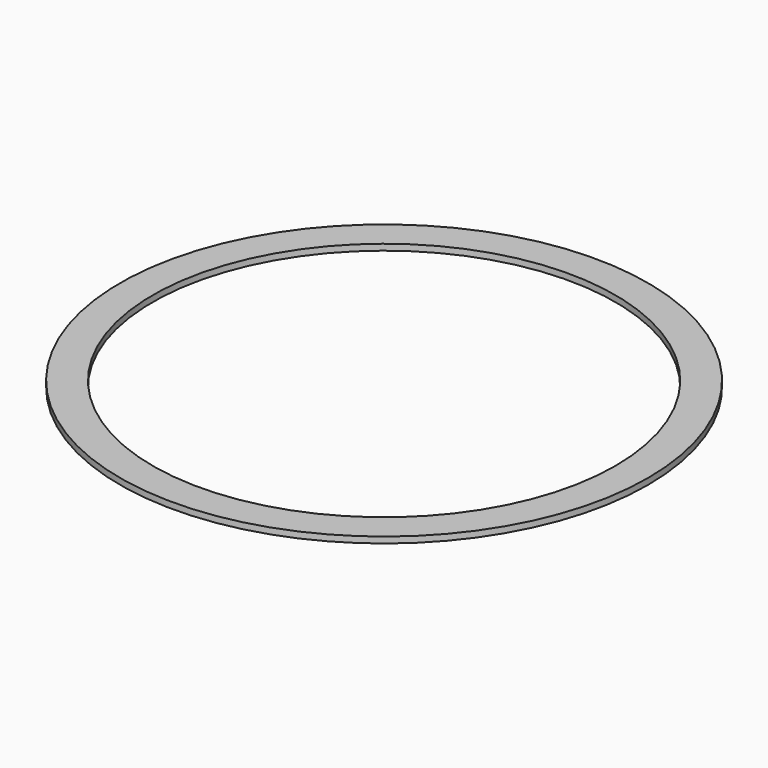
from build123d import *

# Parameters (mm, degrees)
F0_R     = 205.20533
F0_R_2   = 179.80533
F1_DEPTH = 4.7625


# Not quite as in the source:
# - a length typed as a fraction of an inch, garbled in the dataset ("3 / 203.2 mm" for 3/8 in), is restored


with BuildPart() as f1:
    # F0 (on Top) → F1 (new body)
    with BuildSketch(Plane.XY):
        Circle(F0_R)
        Circle(F0_R_2, mode=Mode.SUBTRACT)
    extrude(amount=F1_DEPTH)


solid = f1.part
